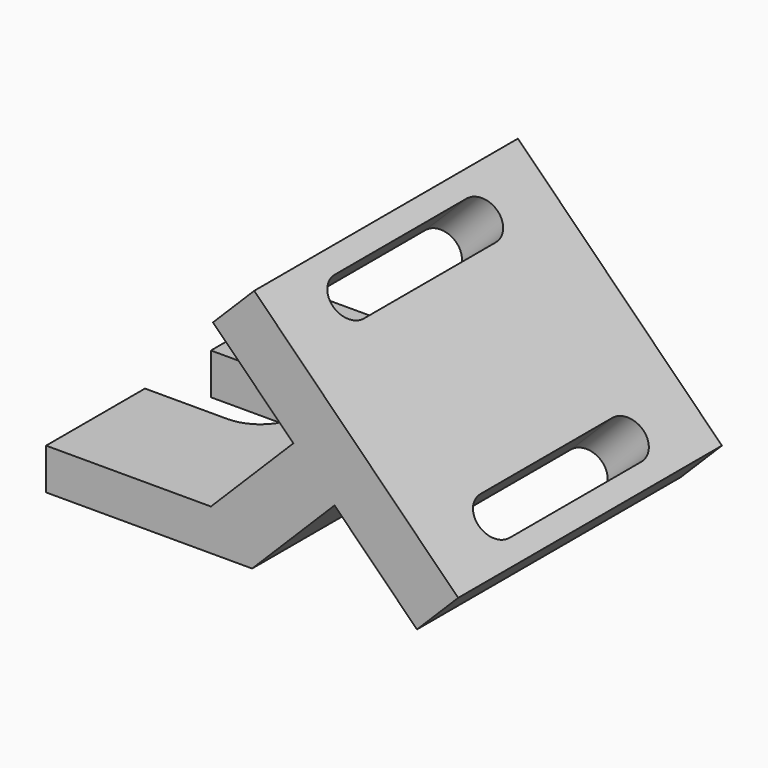
from build123d import *

# Parameters (mm, degrees)
F1_DEPTH = 12.7
F2_SIZE  = 25.39999
F3_DEPTH = 71.8420489686
F4_W     = 203.2
F4_H     = 70.0369336182
F4_H_2   = 71.8420560396
F4_H_3   = 35.9210103421
F5_DEPTH = 35.9156


# Not quite as in the source:
# - a fillet or chamfer is up to 0.001 mm smaller than in the source, because OpenCascade refuses the exact size


with BuildPart() as f1:
    # F0 (on Top) → F1 (new body, symmetric)
    with BuildSketch(Plane.XY):
        with BuildLine():
            Line((0, 76.2), (0, 0))
            Line((0, 0), (127, 0))
            Line((127, 0), (127, 203.2))
            Line((127, 203.2), (0, 203.2))
            Line((0, 203.2), (0, 127))
            Line((0, 127), (50.8, 127))
            ThreePointArc((50.8, 127), (76.2, 101.6), (50.8, 76.2))
            Line((50.8, 76.2), (0, 76.2))
        make_face()
    extrude(amount=F1_DEPTH, both=True)

    # F2 (size 25.4 in the source; OpenCascade refuses exactly that, so slightly less here)
    f2_edges = [f1.edges().sort_by_distance(p)[0] for p in [
        (127, 101.6, 12.7),
    ]]
    chamfer(f2_edges, length=F2_SIZE)

    # F3 (add): a face of the model
    f3_faces = [f1.faces().sort_by_distance(p)[0] for p in [
        (114.300005, 101.6, 5e-06),
    ]]
    extrude(f3_faces, amount=F3_DEPTH)

    # F4 (on face) → F5 (join)
    with BuildSketch(Plane(origin=(107.95, 0, 107.95), x_dir=(0, 1, 0), z_dir=(0.7071067812, 0, 0.7071067812))):
        with Locations((101.6, -27.8433331094)):
            Rectangle(F4_W, F4_H)
        with BuildLine():
            ThreePointArc((50.8, -30.9248663003), (38.1, -18.2248663003), (50.8, -5.5248663003))
            Line((50.8, -5.5248663003), (152.4, -5.5248663003))
            ThreePointArc((152.4, -5.5248663003), (165.1, -18.2248663003), (152.4, -30.9248663003))
            Line((152.4, -30.9248663003), (50.8, -30.9248663003))
        make_face(mode=Mode.SUBTRACT)
        with Locations((101.6, -134.7038382805)):
            Rectangle(F4_W, F4_H_2)
        with BuildLine():
            ThreePointArc((50.8, -157.9248663003), (38.1, -145.2248663003), (50.8, -132.5248663003))
            Line((50.8, -132.5248663003), (152.4, -132.5248663003))
            ThreePointArc((152.4, -132.5248663003), (165.1, -145.2248663003), (152.4, -157.9248663003))
            Line((152.4, -157.9248663003), (50.8, -157.9248663003))
        make_face(mode=Mode.SUBTRACT)
        with Locations((101.6, -80.8223050896)):
            Rectangle(F4_W, F4_H_3)
    extrude(amount=F5_DEPTH)


solid = f1.part
